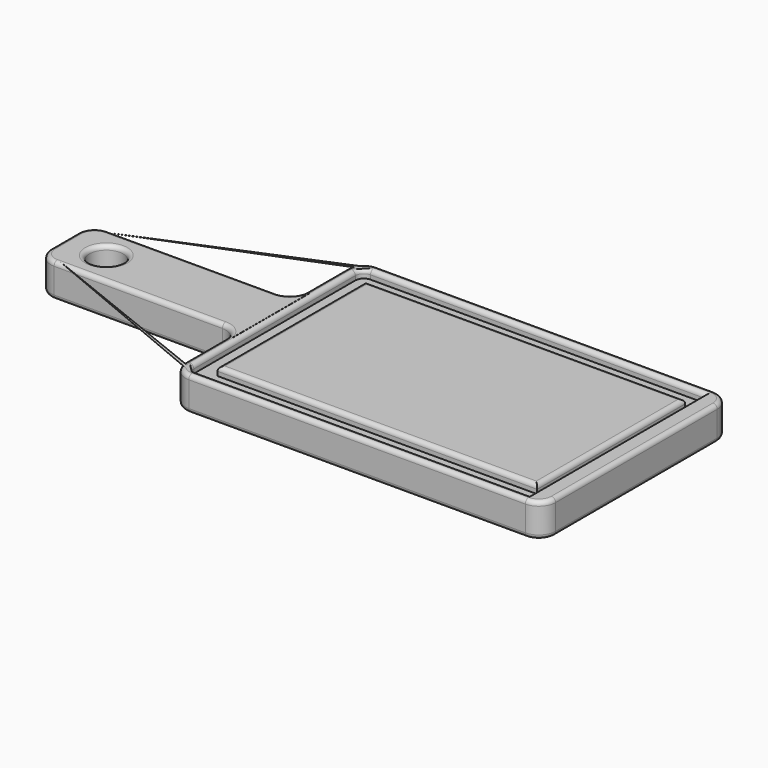
from build123d import *

# Parameters (mm, degrees)
F0_W     = 152.4
F0_H     = 50.8
F1_DEPTH = 25.4
F2_R     = 12.7
F3_DEPTH = 25.4
F5_DEPTH = 6.35
F6_R     = 6.35
F7_R     = 12.7
F8_R     = 3.17499


# Not quite as in the source:
# - a fillet or chamfer is up to 0.001 mm smaller than in the source, because OpenCascade refuses the exact size


with BuildPart() as f1:
    # F0 (on Top) → F1 (new body)
    with BuildSketch(Plane.XY):
        Polygon((0, 63.5), (0, 0), (279.4, 0), (279.4, 177.8), (0, 177.8), (0, 114.3), align=None)
        with Locations((-76.2, 88.9)):
            Rectangle(F0_W, F0_H)
    extrude(amount=F1_DEPTH)

    # F2 (on face) → F3 (cut)
    with BuildSketch(Plane.XY.offset(25.4)):
        with Locations((-120.65, 88.9)):
            Circle(F2_R)
    extrude(amount=-F3_DEPTH, mode=Mode.SUBTRACT)

    # F4 (on face) → F5 (cut)
    with BuildSketch(Plane.XY.offset(25.4)):
        Polygon((273.05, 6.35), (273.05, 171.45), (6.35, 171.45), (6.35, 107.95), (6.35, 69.85), (6.35, 6.35), align=None)
        Polygon((19.05, 107.95), (19.05, 158.75), (260.35, 158.75), (260.35, 19.05), (19.05, 19.05), (19.05, 69.85), align=None, mode=Mode.SUBTRACT)
    extrude(amount=-F5_DEPTH, mode=Mode.SUBTRACT)

    # F6
    f6_edges = [f1.edges().sort_by_distance(p)[0] for p in [
        (6.35, 171.45, 22.225),
        (273.05, 171.45, 22.225),
        (6.35, 6.35, 22.225),
        (273.05, 6.35, 22.225),
    ]]
    fillet(f6_edges, radius=F6_R)

    # F7
    f7_edges = [f1.edges().sort_by_distance(p)[0] for p in [
        (0, 0, 12.7),
        (-152.4, 63.5, 12.7),
        (0, 63.5, 12.7),
        (-152.4, 114.3, 12.7),
        (0, 114.3, 12.7),
        (0, 177.8, 12.7),
        (279.4, 0, 12.7),
        (279.4, 177.8, 12.7),
    ]]
    fillet(f7_edges, radius=F7_R)

    # F8 (radius 3.175 in the source; OpenCascade refuses exactly that, so slightly less here)
    f8_edges = [f1.edges().sort_by_distance(p)[0] for p in [
        (139.7, 19.05, 25.4),
        (19.05, 88.9, 25.4),
        (139.7, 158.75, 25.4),
        (260.35, 88.9, 25.4),
        (0, 31.75, 25.4),
        (-3.719744, 59.780256, 25.4),
        (3.719744, 3.719744, 25.4),
        (-76.2, 63.5, 25.4),
        (139.7, 0, 25.4),
        (-148.680256, 67.219744, 25.4),
        (275.680256, 3.719744, 25.4),
        (-152.4, 88.9, 25.4),
        (279.4, 88.9, 25.4),
        (-148.680256, 110.580256, 25.4),
        (275.680256, 174.080256, 25.4),
        (-76.2, 114.3, 25.4),
        (139.7, 177.8, 25.4),
        (-3.719744, 118.019744, 25.4),
        (3.719744, 174.080256, 25.4),
        (0, 146.05, 25.4),
        (139.7, 6.35, 25.4),
        (8.209872, 8.209872, 25.4),
        (271.190128, 8.209872, 25.4),
        (6.35, 88.9, 25.4),
        (273.05, 88.9, 25.4),
        (8.209872, 169.590128, 25.4),
        (271.190128, 169.590128, 25.4),
        (139.7, 171.45, 25.4),
        (-133.35, 88.9, 25.4),
        (0, 31.75, 0),
        (-3.719744, 59.780256, 0),
        (3.719744, 3.719744, 0),
        (-76.2, 63.5, 0),
        (139.7, 0, 0),
        (-148.680256, 67.219744, 0),
        (275.680256, 3.719744, 0),
        (-152.4, 88.9, 0),
        (279.4, 88.9, 0),
        (-148.680256, 110.580256, 0),
        (275.680256, 174.080256, 0),
        (-76.2, 114.3, 0),
        (139.7, 177.8, 0),
        (-3.719744, 118.019744, 0),
        (3.719744, 174.080256, 0),
        (0, 146.05, 0),
        (-133.35, 88.9, 0),
    ]]
    fillet(f8_edges, radius=F8_R)


solid = f1.part
